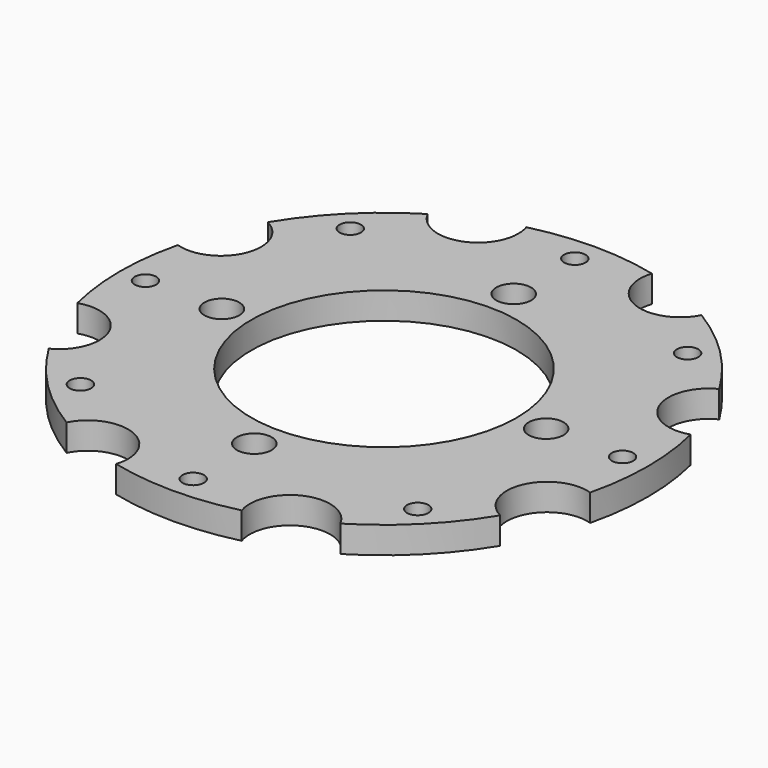
from build123d import *

# Parameters (mm, degrees)
F0_R     = 4
F0_R_2   = 6.5
F0_R_3   = 49.5
F1_DEPTH = 10


# Not quite as in the source:
# - ends of sketch curves that miss each other by under 0.0002 mm in the source are joined


with BuildPart() as f1:
    # F0 (on Top) → F1 (new body)
    with BuildSketch(Plane.XY):
        with BuildLine():
            ThreePointArc((95.6705294551, -23.4392788665), (97.790074014, -11.804720426), (98.5, 0))
            ThreePointArc((98.5, 0), (97.790074014, 11.804720426), (95.6705294551, 23.4392788665))
            ThreePointArc((95.6705294551, 23.4392788665), (77.143947059, 31.9540684018), (84.2233479596, 51.0752010798))
            ThreePointArc((84.2233479596, 51.0752010798), (69.6500179469, 69.6500179469), (51.0752071036, 84.2233531708))
            ThreePointArc((51.0752071036, 84.2233531708), (31.9540684018, 77.143947059), (23.4392785061, 95.6705221617))
            ThreePointArc((23.4392785061, 95.6705221617), (0, 98.5), (-23.4392788665, 95.6705294551))
            ThreePointArc((-23.4392788665, 95.6705294551), (-22.8817314531, 93.3658702171), (-22.69432, 91.00214))
            ThreePointArc((-22.69432, 91.00214), (-34.2095830083, 76.4125338333), (-51.0752010798, 84.2233479596))
            ThreePointArc((-51.0752010798, 84.2233479596), (-69.6500179469, 69.6500179469), (-84.2233531708, 51.0752071036))
            ThreePointArc((-84.2233531708, 51.0752071036), (-78.2216528988, 45.5466540133), (-76.00214, 37.69432))
            ThreePointArc((-76.00214, 37.69432), (-82.1994623513, 25.5488325165), (-95.6705221617, 23.4392785061))
            ThreePointArc((-95.6705221617, 23.4392785061), (-98.5, 0), (-95.6705294551, -23.4392788665))
            ThreePointArc((-95.6705294551, -23.4392788665), (-82.1994623513, -25.5488325165), (-76.00214, -37.69432))
            ThreePointArc((-76.00214, -37.69432), (-78.2216493872, -45.5466482978), (-84.2233479596, -51.0752010798))
            ThreePointArc((-84.2233479596, -51.0752010798), (-69.6500179469, -69.6500179469), (-51.0752071036, -84.2233531708))
            ThreePointArc((-51.0752071036, -84.2233531708), (-34.2095830083, -76.4125338333), (-22.69432, -91.00214))
            ThreePointArc((-22.69432, -91.00214), (-22.8817303816, -93.3658635024), (-23.4392785061, -95.6705221617))
            ThreePointArc((-23.4392785061, -95.6705221617), (0, -98.5), (23.4392788665, -95.6705294551))
            ThreePointArc((23.4392788665, -95.6705294551), (31.9540745992, -77.143944492), (51.0752071429, -84.2233599276))
            ThreePointArc((51.0752071429, -84.2233599276), (69.6500179469, -69.6500179469), (84.2233531708, -51.0752071036))
            ThreePointArc((84.2233531708, -51.0752071036), (77.1439496611, -31.9540621197), (95.6705294551, -23.4392788665))
        make_face()
        with Locations((-62.9325, -62.9325)):
            Circle(F0_R, mode=Mode.SUBTRACT)
        with Locations((0, -89)):
            Circle(F0_R, mode=Mode.SUBTRACT)
        with Locations((0, -60.5)):
            Circle(F0_R_2, mode=Mode.SUBTRACT)
        with Locations((-89, 0)):
            Circle(F0_R, mode=Mode.SUBTRACT)
        with Locations((-60.5, 0)):
            Circle(F0_R_2, mode=Mode.SUBTRACT)
        Circle(F0_R_3, mode=Mode.SUBTRACT)
        with Locations((62.9325, -62.9325)):
            Circle(F0_R, mode=Mode.SUBTRACT)
        with Locations((60.5, 0)):
            Circle(F0_R_2, mode=Mode.SUBTRACT)
        with Locations((89, 0)):
            Circle(F0_R, mode=Mode.SUBTRACT)
        with Locations((-62.9325, 62.9325)):
            Circle(F0_R, mode=Mode.SUBTRACT)
        with Locations((0, 60.5)):
            Circle(F0_R_2, mode=Mode.SUBTRACT)
        with Locations((0, 89)):
            Circle(F0_R, mode=Mode.SUBTRACT)
        with Locations((62.9325, 62.9325)):
            Circle(F0_R, mode=Mode.SUBTRACT)
    extrude(amount=F1_DEPTH)


solid = f1.part
